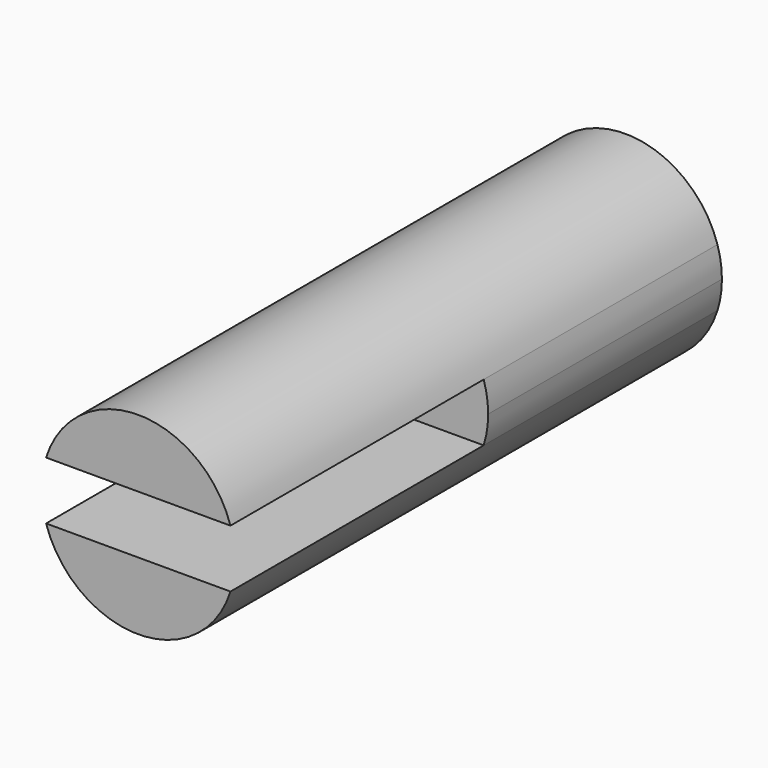
from build123d import *

# Parameters (mm, degrees)
F1_DEPTH = 25
F2_DEPTH = 12


# Not quite as in the source:
# - a feature names something its author has since deleted; it is built from what else it names


with BuildPart() as f1:
    # F0 (on Front) → F1 (new body)
    with BuildSketch(Plane.XZ):
        with BuildLine():
            Line((-44.8163774249, 23.8675290289), (-41.9426736004, 23.8675290289))
            ThreePointArc((-41.9426736004, 23.8675290289), (-45.7285804931, 26.6455290289), (-49.5144873857, 23.8675290289))
            Line((-49.5144873857, 23.8675290289), (-46.6407835612, 23.8675290289))
            ThreePointArc((-46.6407835612, 23.8675290289), (-45.7285804931, 24.1767790289), (-44.8163774249, 23.8675290289))
        make_face()
        with BuildLine():
            Line((-46.6407835612, 23.8675290289), (-44.8163774249, 23.8675290289))
            ThreePointArc((-44.8163774249, 23.8675290289), (-45.7285804931, 24.1767790289), (-46.6407835612, 23.8675290289))
        make_face()
    extrude(amount=F1_DEPTH)



with BuildPart() as f1b:
    # F0 (on Front) → F1, piece 2 (new body)
    with BuildSketch(Plane.XZ):
        with BuildLine():
            ThreePointArc((-49.5144873857, 21.4860290289), (-45.7285804931, 18.7080290289), (-41.9426736004, 21.4860290289))
            Line((-41.9426736004, 21.4860290289), (-44.8163774249, 21.4860290289))
            ThreePointArc((-44.8163774249, 21.4860290289), (-45.7285804931, 21.1767790289), (-46.6407835612, 21.4860290289))
            Line((-46.6407835612, 21.4860290289), (-49.5144873857, 21.4860290289))
        make_face()
        with BuildLine():
            ThreePointArc((-46.6407835612, 21.4860290289), (-45.7285804931, 21.1767790289), (-44.8163774249, 21.4860290289))
            Line((-44.8163774249, 21.4860290289), (-46.6407835612, 21.4860290289))
        make_face()
    extrude(amount=F1_DEPTH)


with BuildPart() as f1_1:
    add(f1.part)

    add(f1b.part)  # F2 merges F1b
    # F0 (on Front) → F2 (join)
    with BuildSketch(Plane.XZ):
        with BuildLine():
            Line((-46.6407835612, 23.8675290289), (-49.5144873857, 23.8675290289))
            ThreePointArc((-49.5144873857, 23.8675290289), (-49.6973304931, 22.6767790289), (-49.5144873857, 21.4860290289))
            Line((-49.5144873857, 21.4860290289), (-46.6407835612, 21.4860290289))
            ThreePointArc((-46.6407835612, 21.4860290289), (-47.2285804931, 22.6767790289), (-46.6407835612, 23.8675290289))
        make_face()
        with BuildLine():
            ThreePointArc((-41.9426736004, 21.4860290289), (-41.8058075872, 22.0744259007), (-41.7598304931, 22.6767790289))
            ThreePointArc((-41.7598304931, 22.6767790289), (-41.8058075872, 23.2791321571), (-41.9426736004, 23.8675290289))
            Line((-41.9426736004, 23.8675290289), (-44.8163774249, 23.8675290289))
            ThreePointArc((-44.8163774249, 23.8675290289), (-44.3835331701, 23.3407426566), (-44.2285804931, 22.6767790289))
            ThreePointArc((-44.2285804931, 22.6767790289), (-44.3835331701, 22.0128154012), (-44.8163774249, 21.4860290289))
            Line((-44.8163774249, 21.4860290289), (-41.9426736004, 21.4860290289))
        make_face()
    extrude(amount=F2_DEPTH)


solid = f1_1.part
